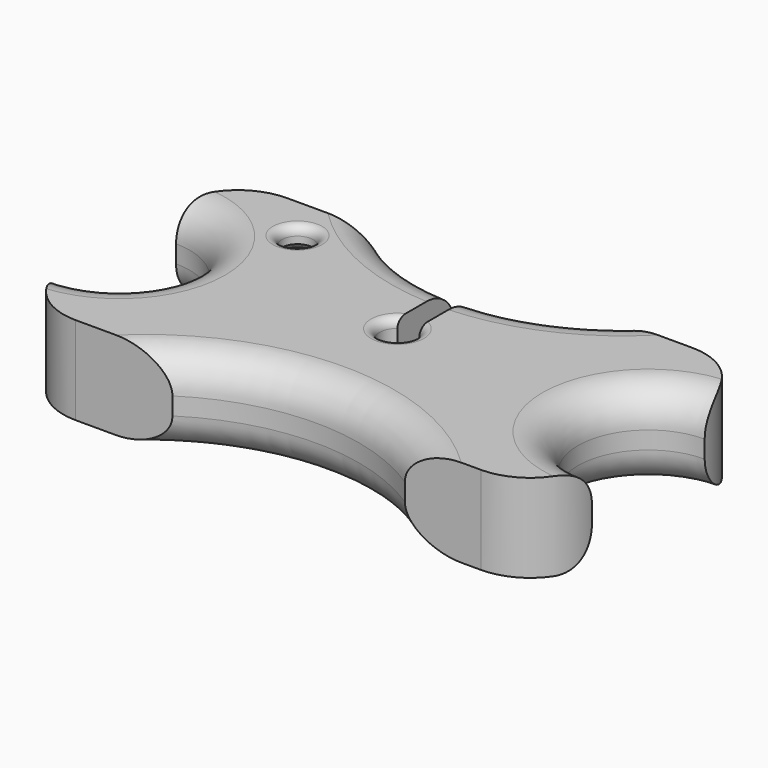
from build123d import *

# Parameters (mm, degrees)
F1_DEPTH  = 10
F2_R      = 4
F3_R      = 2.5
F4_DEPTH  = 7.5
F5_R      = 1.8
F6_DEPTH  = 29.012279585
F7_R      = 1
F8_SIZE   = 0.69999
F10_DEPTH = 25
F11_R     = 1


# Not quite as in the source:
# - a fillet or chamfer is up to 0.001 mm smaller than in the source, because OpenCascade refuses the exact size


with BuildPart() as f1:
    # F0 (on Top) → F1 (new body)
    with BuildSketch(Plane.XY):
        with BuildLine():
            Line((3.8354769349, 19.5987266302), (-7.0263877602, 19.5987266302))
            ThreePointArc((-7.0263877602, 19.5987266302), (-11.9761352285, 17.5484740985), (-14.0263877602, 12.5987266302))
            ThreePointArc((-14.0263877602, 12.5987266302), (-6.0681101368, 4.5987266302), (-14.0263877602, -3.4012733698))
            ThreePointArc((-14.0263877602, -3.4012733698), (-11.9761352285, -8.3510208381), (-7.0263877602, -10.4012733698))
            Line((-7.0263877602, -10.4012733698), (3.9582140744, -10.4012733698))
            ThreePointArc((3.9582140744, -10.4012733698), (17.1527732164, -6.4998852769), (30.3473323584, -10.4012733698))
            Line((30.3473323584, -10.4012733698), (38.9736122398, -10.4012733698))
            ThreePointArc((38.9736122398, -10.4012733698), (43.9233597081, -8.3510208381), (45.9736122398, -3.4012733698))
            ThreePointArc((45.9736122398, -3.4012733698), (37.9736122398, 4.5987266302), (45.9736122398, 12.5987266302))
            ThreePointArc((45.9736122398, 12.5987266302), (43.9233597081, 17.5484740985), (38.9736122398, 19.5987266302))
            Line((38.9736122398, 19.5987266302), (28.8130864501, 19.5987266302))
            ThreePointArc((28.8130864501, 19.5987266302), (16.3242816925, 15.7745774939), (3.8354769349, 19.5987266302))
        make_face()
    extrude(amount=F1_DEPTH)

    # F2
    f2_edges = [f1.edges().sort_by_distance(p)[0] for p in [
        (17.152773, -6.499885, 10),
        (-6.06811, 4.598727, 10),
        (16.324282, 15.774577, 10),
        (37.973612, 4.598727, 10),
        (-6.06811, 4.598727, 0),
        (17.152773, -6.499885, 0),
        (16.324282, 15.774577, 0),
        (37.973612, 4.598727, 0),
    ]]
    fillet(f2_edges, radius=F2_R)

    # F3 (on Top) → F4 (cut)
    with BuildSketch(Plane.XY):
        with Locations((-1.8226802303, 14.5681592802)):
            Circle(F3_R)
    extrude(amount=F4_DEPTH, mode=Mode.SUBTRACT)

    # F5 (on Top) → F6 (cut)
    with BuildSketch(Plane.XY):
        with Locations((-1.8226802303, 14.5681592802)):
            Circle(F5_R)
    extrude(amount=F6_DEPTH, mode=Mode.SUBTRACT)

    # F7
    f7_edges = [f1.edges().sort_by_distance(p)[0] for p in [
        (-4.32268, 14.568159, 0),
        (-3.62268, 14.568159, 10),
    ]]
    fillet(f7_edges, radius=F7_R)

    # F8 (size 0.7 in the source; OpenCascade refuses exactly that, so slightly less here)
    f8_edges = [f1.edges().sort_by_distance(p)[0] for p in [
        (-3.62268, 14.568159, 7.5),
    ]]
    chamfer(f8_edges, length=F8_SIZE)

    # F9 (on Top) → F10 (cut)
    with BuildSketch(Plane.XY):
        with BuildLine():
            Line((17.52821289, 16.1215772422), (15.02821289, 16.1215772422))
            Line((15.02821289, 16.1215772422), (15.02821289, 7.6828267418))
            ThreePointArc((15.02821289, 7.6828267418), (16.27821289, 4.1215772422), (17.52821289, 7.6828267418))
            Line((17.52821289, 7.6828267418), (17.52821289, 16.1215772422))
        make_face()
    extrude(amount=F10_DEPTH, mode=Mode.SUBTRACT)

    # F11
    f11_edges = [f1.edges().sort_by_distance(p)[0] for p in [
        (16.278213, 4.121577, 10),
        (16.278213, 4.121577, 0),
    ]]
    fillet(f11_edges, radius=F11_R)


solid = f1.part
